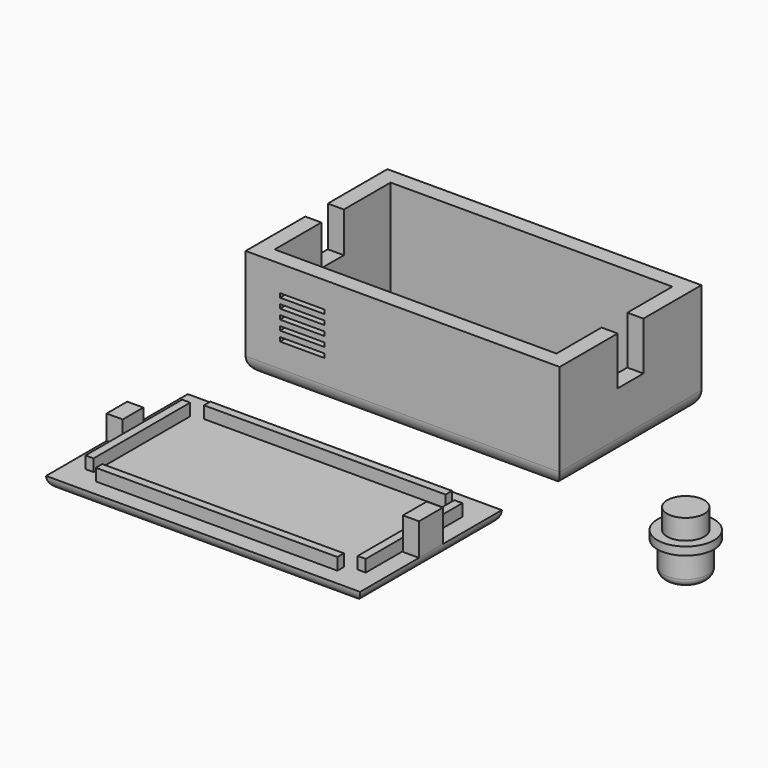
from build123d import *

# Parameters (mm, degrees)
F0_W      = 35
F0_H      = 18
F1_DEPTH  = 1.5
F0_W_2    = 39
F0_H_2    = 22
F2_DEPTH  = 13.5
F3_D      = 3.3
F3_DEPTH  = 5
F3_TIP    = 0.9914200214
F5_D      = 6
F5_DEPTH  = 5
F5_TIP    = 1.8025818571
F7_R      = 2.3
F8_DEPTH  = 7.5
F7_R_2    = 2.75
F9_DEPTH  = 4
F10_R     = 1
F11_R     = 3.5143854074
F11_R_2   = 2.75
F11_R_3   = 2.3
F12_DEPTH = 1
F14_W     = 6
F14_H     = 6
F15_DEPTH = 0.75
F16_W     = 3.5
F16_H     = 5
F17_DEPTH = 5
F18_W     = 1
F18_H     = 15
F18_W_2   = 30
F18_H_2   = 1
F19_DEPTH = 1.5
F20_DEPTH = 3
F6_W      = 4
F6_H      = 2
F6_H_2    = 4
F21_DEPTH = 5
F18_W_3   = 2
F18_H_3   = 3.7
F22_DEPTH = 5.5
F23_W     = 5.5
F23_H     = 0.5
F24_DEPTH = 5
F18_H_4   = 3.2
F25_DEPTH = 4.5
F26_R     = 2
F27_R     = 1.49999


# Not quite as in the source:
# - a fillet or chamfer is up to 0.001 mm smaller than in the source, because OpenCascade refuses the exact size
# - a feature names something its author has since deleted; it is built from what else it names


with BuildPart() as f1:
    # F0 (on Top) → F1 (new body)
    with BuildSketch(Plane.XY):
        Rectangle(F0_W, F0_H)
    extrude(amount=F1_DEPTH)

    # F0 (on Top) → F2 (join)
    with BuildSketch(Plane.XY):
        Rectangle(F0_W_2, F0_H_2)
        Rectangle(F0_W, F0_H, mode=Mode.SUBTRACT)
    extrude(amount=F2_DEPTH)

    # F3
    with Locations(Plane(origin=(0, 0, 0), x_dir=(1, 0, 0), z_dir=(0, 0, -1))):
        with Locations((8.3, 4)):
            Hole(F3_D / 2, depth=F3_DEPTH)
            with Locations((0, 0, -(F3_DEPTH + F3_TIP / 2))):  # 118° drill point
                Cone(0, F3_D / 2, F3_TIP, mode=Mode.SUBTRACT)

    # F5
    with Locations(Plane(origin=(0, 0, 0), x_dir=(1, 0, 0), z_dir=(0, 0, -1))):
        with Locations((8.3, -2.5)):
            Hole(F5_D / 2, depth=F5_DEPTH)
            with Locations((0, 0, -(F5_DEPTH + F5_TIP / 2))):  # 118° drill point
                Cone(0, F5_D / 2, F5_TIP, mode=Mode.SUBTRACT)

    # F14 (on offset) → F15 (cut, symmetric)
    with BuildSketch(Plane.XZ.offset(9)):
        with Locations((-12.5, 7.7)):
            Rectangle(F14_W, F14_H)
    extrude(amount=F15_DEPTH, both=True, mode=Mode.SUBTRACT)

    # F16 (on face) → F17 (cut)
    with BuildSketch(Plane(origin=(-19.5, 0, 0), x_dir=(0, -1, 0), z_dir=(-1, 0, 0))):
        with Locations((0, 11)):
            Rectangle(F16_W, F16_H)
    extrude(amount=-F17_DEPTH, mode=Mode.SUBTRACT)

    # F6 (on face) → F21 (cut)
    with BuildSketch(Plane.YZ.offset(19.5)):
        with Locations((0, 8.5)):
            Rectangle(F6_W, F6_H)
        with Locations((0, 11.5)):
            Rectangle(F6_W, F6_H_2)
    extrude(amount=-F21_DEPTH, mode=Mode.SUBTRACT)

    # F23 (on face) → F24 (cut)
    with BuildSketch(Plane.XZ.offset(11)):
        with Locations((-12.4855237082, 5.2288122736)):
            Rectangle(F23_W, F23_H)
        with Locations((-12.4855237082, 6.4288122736)):
            Rectangle(F23_W, F23_H)
        with Locations((-12.4855237082, 7.6288122736)):
            Rectangle(F23_W, F23_H)
        with Locations((-12.4855237082, 8.8288122736)):
            Rectangle(F23_W, F23_H)
        with Locations((-12.4855237082, 10.0288122736)):
            Rectangle(F23_W, F23_H)
    extrude(amount=-F24_DEPTH, mode=Mode.SUBTRACT)

    # F26
    f26_edges = [f1.edges().sort_by_distance(p)[0] for p in [
        (0, -11, 0),
        (-19.5, 0, 0),
        (19.5, 0, 0),
        (0, 11, 0),
    ]]
    fillet(f26_edges, radius=F26_R)


with BuildPart() as f8:
    # F7 (on Top) → F8 (new body)
    with BuildSketch(Plane.XY):
        with Locations((40.214437741, -17.3225737277)):
            Circle(F7_R)
    extrude(amount=F8_DEPTH)

    # F7 (on Top) → F9 (join)
    with BuildSketch(Plane.XY):
        with Locations((40.214437741, -17.3225737277)):
            Circle(F7_R_2)
        with Locations((40.214437741, -17.3225737277)):
            Circle(F7_R, mode=Mode.SUBTRACT)
    extrude(amount=F9_DEPTH)

    # F10
    f10_edges = [f8.edges().sort_by_distance(p)[0] for p in [
        (37.464438, -17.322574, 0),
    ]]
    fillet(f10_edges, radius=F10_R)

    # F11 (on face) → F12 (join)
    with BuildSketch(Plane.XY.offset(4)):
        with Locations((40.214437741, -17.3225737277)):
            Circle(F11_R)
        with Locations((40.214437741, -17.3225737277)):
            Circle(F11_R_2, mode=Mode.SUBTRACT)
        with Locations((40.214437741, -17.3225737277)):
            Circle(F11_R_2)
        with Locations((40.214437741, -17.3225737277)):
            Circle(F11_R_3, mode=Mode.SUBTRACT)
    extrude(amount=F12_DEPTH)


with BuildPart() as f19:
    # F18 (on Top) → F19 (new body)
    with BuildSketch(Plane.XY):
        Polygon((-19.5, -41.9833288193), (19.5, -41.9833288193), (19.5, -32.8333288193), (17.5, -32.8333288193), (17.5, -29.1333288193), (19.5, -29.1333288193), (19.5, -19.9833288193), (-19.5, -19.9833288193), (-19.5, -29.3833288193), (-17.5, -29.3833288193), (-17.5, -32.5833288193), (-19.5, -32.5833288193), align=None)
        with Locations((-16.9, -30.9833288193)):
            Rectangle(F18_W, F18_H, mode=Mode.SUBTRACT)
        with Locations((0, -39.3833288193)):
            Rectangle(F18_W_2, F18_H_2, mode=Mode.SUBTRACT)
        with Locations((16.9, -30.9833288193)):
            Rectangle(F18_W, F18_H, mode=Mode.SUBTRACT)
        with Locations((0, -22.5915573537)):
            Rectangle(F18_W_2, F18_H_2, mode=Mode.SUBTRACT)
    extrude(amount=F19_DEPTH)

    # F18 (on Top) → F20 (join)
    with BuildSketch(Plane.XY):
        with Locations((0, -22.5915573537)):
            Rectangle(F18_W_2, F18_H_2)
        with Locations((-16.9, -30.9833288193)):
            Rectangle(F18_W, F18_H)
        with Locations((0, -39.3833288193)):
            Rectangle(F18_W_2, F18_H_2)
        with Locations((16.9, -30.9833288193)):
            Rectangle(F18_W, F18_H)
    extrude(amount=F20_DEPTH)

    # F18 (on Top) → F22 (join)
    with BuildSketch(Plane.XY):
        with Locations((18.5, -30.9833288193)):
            Rectangle(F18_W_3, F18_H_3)
    extrude(amount=F22_DEPTH)

    # F18 (on Top) → F25 (join)
    with BuildSketch(Plane.XY):
        with Locations((-18.5, -30.9833288193)):
            Rectangle(F18_W_3, F18_H_4)
    extrude(amount=F25_DEPTH)

    # F27 (radius 1.5 in the source; OpenCascade refuses exactly that, so slightly less here)
    f27_edges = [f19.edges().sort_by_distance(p)[0] for p in [
        (19.5, -30.983329, 0),
        (0, -19.983329, 0),
        (-19.5, -30.983329, 0),
        (0, -41.983329, 0),
    ]]
    fillet(f27_edges, radius=F27_R)


solid = Compound([f1.part, f8.part, f19.part])
